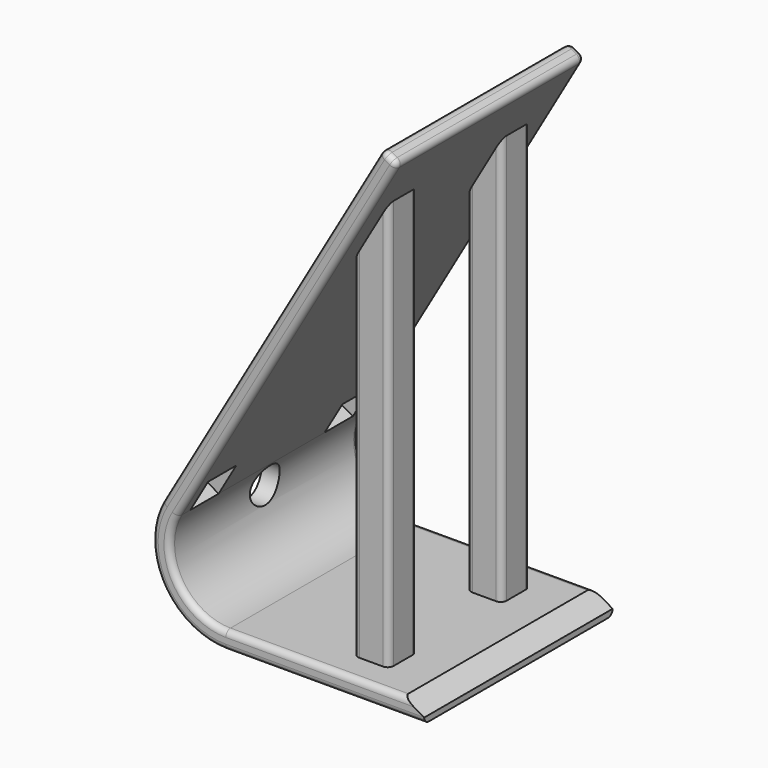
from build123d import *

# Parameters (mm, degrees)
F1_DEPTH     = 80
F2_W         = 12
F2_H         = 12
F5_D         = 12.5
F6_W         = 12
F6_H         = 12
F7_DEPTH     = 10
F8_TEXT_SIZE = 18.1944444444
F9_DEPTH     = 3
F10_R        = 2
F11_R        = 2
F12_T1_DEPTH = 112.219200565


# Not quite as in the source:
# - a fillet or chamfer that OpenCascade refuses, or shapes differently, is made with other operations: its cross-section is extruded or revolved along the edge and cut away or added
# - Text() gives the source's letters only with a copy of the font that has no kerning and outlines rounded to 1/6400 em; it was checked with that copy


with BuildPart() as f1:
    # F0 (on Front) → F1 (new body)
    with BuildSketch(Plane.XZ):
        with BuildLine():
            Line((14.8157308908, -45.5832920319), (82.1650957962, -45.5832920319))
            Line((82.1650957962, -45.5832920319), (82.1650957962, -39.5832920319))
            Line((82.1650957962, -39.5832920319), (14.8157308908, -39.5832920319))
            ThreePointArc((14.8157308908, -39.5832920319), (-1.6387517811, -30.0832920319), (-1.6387517811, -11.0832920319))
            Line((-1.6387517811, -11.0832920319), (73.1650957962, 118.4807725736))
            Line((73.1650957962, 118.4807725736), (67.9689433735, 121.4807725736))
            Line((67.9689433735, 121.4807725736), (-6.8349042038, -8.0832920319))
            ThreePointArc((-6.8349042038, -8.0832920319), (-6.8349042038, -33.0832920319), (14.8157308908, -45.5832920319))
        make_face()
    extrude(amount=F1_DEPTH)

    # F2 (on face) → F3 (join, up to the next surface of F1)
    with BuildSketch(Plane.XY.offset(-39.5832920319)):
        with Locations((56.1650957962, -16)):
            Rectangle(F2_W, F2_H)
        with Locations((56.1650957962, -64)):
            Rectangle(F2_W, F2_H)
    extrude(until=Until.NEXT)

    # F5 (through all)
    with Locations(Plane.YZ):
        with Locations((-40, -18.0832920319)):
            Hole(F5_D / 2)

    # F6 (on face) → F7 (cut)
    with BuildSketch(Plane(origin=(-1.6260100299, 0, 0.9387773285), x_dir=(0, -1, 0), z_dir=(-0.8660254038, 0, 0.5))):
        with Locations((11.5, -4.4177883477)):
            Rectangle(F6_W, F6_H)
        with Locations((68.5, -4.4177883477)):
            Rectangle(F6_W, F6_H)
    extrude(amount=-F7_DEPTH, mode=Mode.SUBTRACT)

    # F8 (on face) → F9 (cut)
    with BuildSketch(Plane(origin=(-1.6260100299, 0, 0.9387773285), x_dir=(0, -1, 0), z_dir=(-0.8660254038, 0, 0.5))):
        with Locations((1.668, 106.0899068068)):
            Text('ROBERT', F8_TEXT_SIZE, font='Arimo', text_align=(TextAlign.LEFT, TextAlign.BOTTOM))
    extrude(amount=-F9_DEPTH, mode=Mode.SUBTRACT)

    # F10
    f10_edges = [f1.edges().sort_by_distance(p)[0] for p in [
        (73.165096, -40, 118.480773),
        (67.968943, -40, 121.480773),
        (62.165096, -10, 29.922461),
        (50.165096, -10, 19.530156),
        (62.165096, -22, 29.922461),
        (50.165096, -22, 19.530156),
        (62.165096, -58, 29.922461),
        (62.165096, -70, 29.922461),
        (50.165096, -70, 19.530156),
        (50.165096, -58, 19.530156),
    ]]
    fillet(f10_edges, radius=F10_R)

    # F11
    f11_edges = [f1.edges().sort_by_distance(p)[0] for p in [
        (30.06702, 0, 55.832715),
        (35.263172, 0, 52.832715),
        (-1.638752, 0, -30.083292),
        (48.490413, 0, -39.583292),
        (48.490413, 0, -45.583292),
        (-6.834904, 0, -33.083292),
        (35.263172, -80, 52.832715),
        (30.06702, -80, 55.832715),
        (-6.834904, -80, -33.083292),
        (48.490413, -80, -39.583292),
        (48.490413, -80, -45.583292),
        (-1.638752, -80, -30.083292),
        (70.56702, 0, 119.980773),
        (70.56702, -80, 119.980773),
        (72.364897, 0, 118.26636),
        (68.183356, 0, 120.680573),
        (72.364897, -80, 118.26636),
        (68.183356, -80, 120.680573),
    ]]
    fillet(f11_edges, radius=F11_R)

    # F12: chamfer of 7 x 4.0414518843 on 1 edges, made by hand

    # F12_s2 → F12_t1 (cut)
    with BuildSketch(Plane.XZ.offset(-16.1096002825)):
        Polygon((82.1650957962, -43.6247439162), (75.1650957962, -39.5832920319), (82.1650957962, -39.5832920319), align=None)
    extrude(amount=F12_T1_DEPTH, mode=Mode.SUBTRACT)


solid = f1.part
